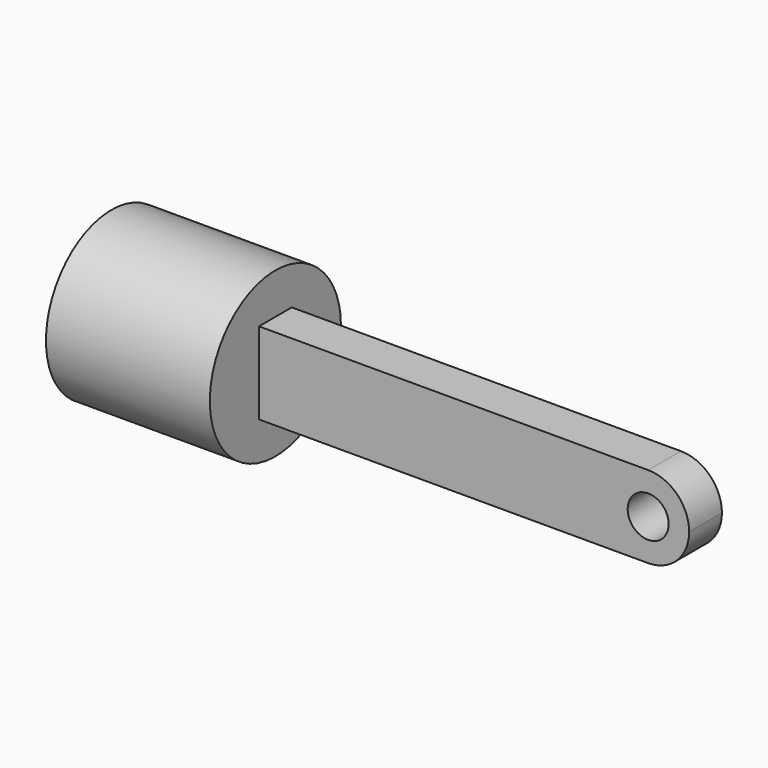
from build123d import *

# Parameters (mm, degrees)
F0_R     = 25.4
F1_DEPTH = 50.8
F2_W     = 12.7
F2_H     = 25.4
F3_DEPTH = 133.35
F4_R     = 12.69999
F5_R     = 6.35
F6_DEPTH = 31.751


# Not quite as in the source:
# - a fillet or chamfer is up to 0.001 mm smaller than in the source, because OpenCascade refuses the exact size


with BuildPart() as f1:
    # F0 (on Right) → F1 (new body)
    with BuildSketch(Plane.YZ):
        Circle(F0_R)
    extrude(amount=-F1_DEPTH)

    # F2 (on face) → F3 (join)
    with BuildSketch(Plane.YZ):
        Rectangle(F2_W, F2_H)
    extrude(amount=F3_DEPTH)

    # F4 (radius 12.7 in the source; OpenCascade refuses exactly that, so slightly less here)
    f4_edges = [f1.edges().sort_by_distance(p)[0] for p in [
        (133.35, 0, 12.7),
        (133.35, 0, -12.7),
    ]]
    fillet(f4_edges, radius=F4_R)

    # F5 (on face) → F6 (cut, through all)
    with BuildSketch(Plane.XZ.offset(6.35)):
        with Locations((120.65, 0)):
            Circle(F5_R)
    extrude(amount=-F6_DEPTH, mode=Mode.SUBTRACT)


solid = f1.part
